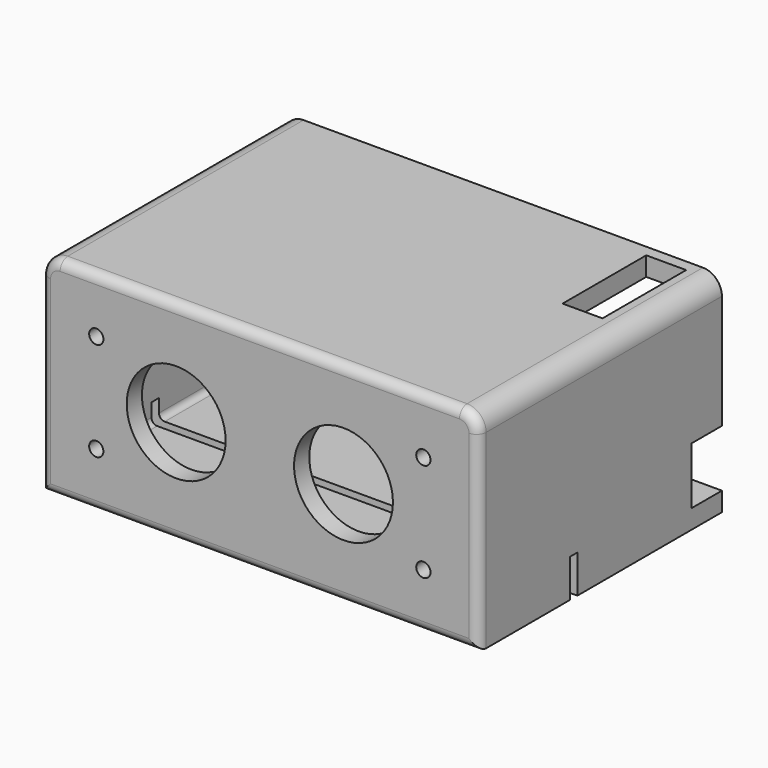
from build123d import *

# Parameters (mm, degrees)
F0_W        = 105
F0_H        = 45
F0_R        = 1.875
F0_R_2      = 13
F1_DEPTH    = 5
F2_W        = 115
F2_H        = 55
F2_W_2      = 105
F2_H_2      = 4.9815587699
F3_DEPTH    = 80
F4_W        = 2.5
F4_H        = 10
F5_DEPTH    = 115.001
F6_R        = 2.5
F7_T1_DEPTH = 92.5
F7_T4_ANGLE = 90
F7_T6_ANGLE = 90
F8_W        = 10.5
F8_H        = 27.5
F9_DEPTH    = 5
F10_W       = 10
F10_H       = 15
F11_DEPTH   = 5.001
F12_R       = 1.5


# Not quite as in the source:
# - a fillet or chamfer that OpenCascade refuses, or shapes differently, is made with other operations: its cross-section is extruded or revolved along the edge and cut away or added


with BuildPart() as f1:
    # F0 (on Front) → F1 (new body)
    with BuildSketch(Plane.XZ):
        Rectangle(F0_W, F0_H)
        with Locations((-43, -13)):
            Circle(F0_R, mode=Mode.SUBTRACT)
        with Locations((43, -13)):
            Circle(F0_R, mode=Mode.SUBTRACT)
        with Locations((-22, 0)):
            Circle(F0_R_2, mode=Mode.SUBTRACT)
        with Locations((-43, 13)):
            Circle(F0_R, mode=Mode.SUBTRACT)
        with Locations((22, 0)):
            Circle(F0_R_2, mode=Mode.SUBTRACT)
        with Locations((43, 13)):
            Circle(F0_R, mode=Mode.SUBTRACT)
    extrude(amount=F1_DEPTH)

    # F2 (on face) → F3 (join)
    with BuildSketch(Plane.XZ.offset(5)):
        Rectangle(F2_W, F2_H)
        Polygon((-52.5, -22.5), (-52.5, 22.5), (52.5, 22.5), (52.5, -22.5), (52.5, -27.4815587699), (-52.5, -27.4815587699), align=None, mode=Mode.SUBTRACT)
        with Locations((0, -24.990779385)):
            Rectangle(F2_W_2, F2_H_2)
    extrude(amount=-F3_DEPTH)

    # F4 (on face) → F5 (cut, through all)
    with BuildSketch(Plane.YZ.offset(57.5)):
        with Locations((26.25, -22.5)):
            Rectangle(F4_W, F4_H)
    extrude(amount=-F5_DEPTH, mode=Mode.SUBTRACT)

    # F6
    f6_edges = [f1.edges().sort_by_distance(p)[0] for p in [
        (0, -5, 27.5),
        (-57.5, -5, 0),
        (0, -5, -27.5),
        (57.5, -5, 0),
    ]]
    fillet(f6_edges, radius=F6_R)

    # F7: fillet of radius 5 on 2 edges, made by hand

    # F7_s2 → F7_t1 (cut)
    with BuildSketch(Plane.XZ.offset(-87.5)):
        with BuildLine():
            ThreePointArc((-52.5, 27.5), (-56.0355339059, 26.0355339059), (-57.5, 22.5))
            Line((-57.5, 22.5), (-57.5, 27.5))
            Line((-57.5, 27.5), (-52.5, 27.5))
        make_face()
        with BuildLine():
            ThreePointArc((52.5, 27.5), (56.0355339059, 26.0355339059), (57.5, 22.5))
            Line((57.5, 22.5), (57.5, 27.5))
            Line((57.5, 27.5), (52.5, 27.5))
        make_face()
    extrude(amount=F7_T1_DEPTH, mode=Mode.SUBTRACT)

    # F7_s3 → F7_t4 (revolve, cut)
    with BuildSketch(Plane.XY.offset(22.5)):
        with BuildLine():
            ThreePointArc((55, -5), (56.767766953, -4.267766953), (57.5, -2.5))
            Line((57.5, -2.5), (57.5, -5))
            Line((57.5, -5), (55, -5))
        make_face()
    revolve(axis=Axis((52.5, -5, 22.5), (0, -1, 0)), revolution_arc=F7_T4_ANGLE, mode=Mode.SUBTRACT)

    # F7_s5 → F7_t6 (revolve, cut)
    with BuildSketch(Plane.YZ.offset(-52.5)):
        with BuildLine():
            ThreePointArc((-5, 25), (-4.267766953, 26.767766953), (-2.5, 27.5))
            Line((-2.5, 27.5), (-5, 27.5))
            Line((-5, 27.5), (-5, 25))
        make_face()
    revolve(axis=Axis((-52.5, -5, 22.5), (0, -1, 0)), revolution_arc=F7_T6_ANGLE, mode=Mode.SUBTRACT)

    # F8 (on face) → F9 (cut, through all)
    with BuildSketch(Plane.XY.offset(27.5)):
        with Locations((45.25, 58.25)):
            Rectangle(F8_W, F8_H)
    extrude(amount=-F9_DEPTH, mode=Mode.SUBTRACT)

    # F10 (on face) → F11 (cut, through all)
    with BuildSketch(Plane(origin=(52.5, 0, 0), x_dir=(0, -1, 0), z_dir=(-1, 0, 0))):
        with Locations((-70, -15)):
            Rectangle(F10_W, F10_H)
    extrude(amount=-F11_DEPTH, mode=Mode.SUBTRACT)

    # F12
    f12_edges = [f1.edges().sort_by_distance(p)[0] for p in [
        (0, 0, -22.5),
        (52.5, 0, 0),
        (0, 0, 22.5),
        (-52.5, 0, 0),
        (-52.5, 37.5, 22.5),
        (52.5, 37.5, 22.5),
        (52.5, 12.5, -22.5),
        (52.5, 46.25, -22.5),
        (-52.5, 12.5, -22.5),
        (-52.5, 51.25, -22.5),
    ]]
    fillet(f12_edges, radius=F12_R)


solid = f1.part
